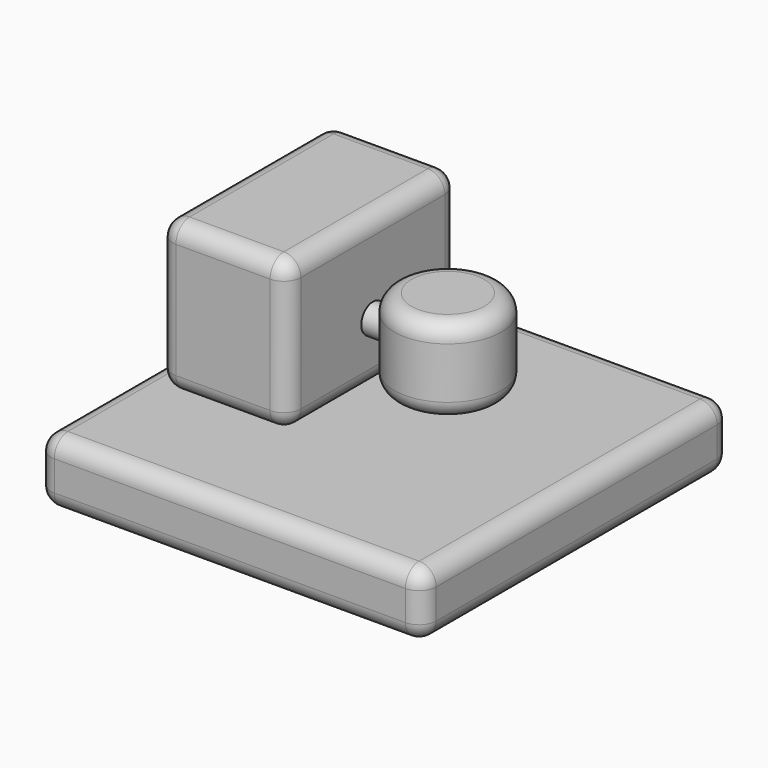
from build123d import *

# Parameters (mm, degrees)
F1_DEPTH      = 57.15
F2_DEPTH      = 57.15
F3_DEPTH      = 31.75
F4_DEPTH      = 31.75
F0_W          = 15.875
F0_H          = 25.4
F6_DEPTH      = 12.7
F7_DEPTH      = 12.7
F0_W_2        = 6.35
F0_H_2        = 4.318
F9_R          = 5.08
F10_R         = 5.08
F11_R         = 5.08
F12_R         = 5.08
F13_R         = 5.08
F13_2_R       = 5.08
F14_R         = 5.08
F15_R         = 5.08
F15_2_R       = 5.08
F16_R         = 5.08
F17_R         = 5.08
F18_R         = 5.08
F19_R         = 5.08
F20_T1_DEPTH  = 53.34
F20_S5_W      = 5.08
F20_S5_H      = 5.08
F20_T6_DEPTH  = 5.08
F20_S11_W     = 5.08
F20_S11_H     = 5.08
F20_T12_DEPTH = 5.08
F20_S17_W     = 5.08
F20_S17_H     = 5.08
F20_T18_DEPTH = 5.08
F20_S23_W     = 5.08
F20_S23_H     = 5.08
F20_T24_DEPTH = 5.08
F21_T1_DEPTH  = 53.34
F21_S5_W      = 5.08
F21_S5_H      = 5.08
F21_T6_DEPTH  = 5.08
F21_S11_W     = 5.08
F21_S11_H     = 5.08
F21_T12_DEPTH = 5.08
F21_S17_W     = 5.08
F21_S17_H     = 5.08
F21_T18_DEPTH = 5.08
F21_S23_W     = 5.08
F21_S23_H     = 5.08
F21_T24_DEPTH = 5.08


# Not quite as in the source:
# - a fillet or chamfer that OpenCascade refuses, or shapes differently, is made with other operations: its cross-section is extruded or revolved along the edge and cut away or added


with BuildPart() as f1:
    # F0 (on Front) → F1 (new body)
    with BuildSketch(Plane.XZ):
        Polygon((57.15, -57.15), (57.15, -38.1), (-22.337236915, -38.1), (-57.15, -38.1), (-57.15, -57.15), align=None)
    extrude(amount=F1_DEPTH)

    # F2 (add): a face of the model
    f2_faces = [f1.faces().sort_by_distance(p)[0] for p in [
        (0, 0, -47.625),
    ]]
    extrude(f2_faces, amount=F2_DEPTH)

    # F9
    f9_edges = [f1.edges().sort_by_distance(p)[0] for p in [
        (0, -57.15, -38.1),
    ]]
    fillet(f9_edges, radius=F9_R)

    # F10
    f10_edges = [f1.edges().sort_by_distance(p)[0] for p in [
        (-57.15, -57.15, -50.165),
    ]]
    fillet(f10_edges, radius=F10_R)

    # F11
    f11_edges = [f1.edges().sort_by_distance(p)[0] for p in [
        (2.54, -57.15, -57.15),
    ]]
    fillet(f11_edges, radius=F11_R)

    # F12
    f12_edges = [f1.edges().sort_by_distance(p)[0] for p in [
        (57.15, -57.15, -47.625),
    ]]
    fillet(f12_edges, radius=F12_R)

    # F14
    f14_edges = [f1.edges().sort_by_distance(p)[0] for p in [
        (0, 57.15, -38.1),
    ]]
    fillet(f14_edges, radius=F14_R)


with BuildPart() as f3:
    # F0 (on Front) → F3 (new body)
    with BuildSketch(Plane.XZ):
        Polygon((-41.387236915, -31.75), (-22.337236915, -31.75), (-3.287236915, -31.75), (-3.287236915, -18.161), (-3.287236915, -13.843), (-3.287236915, -9.525), (-3.287236915, 12.7), (-41.387236915, 12.7), (-41.387236915, -9.525), align=None)
    extrude(amount=F3_DEPTH)

    # F0 (on Front) → F4 (join)
    with BuildSketch(Plane.XZ):
        Polygon((-41.387236915, -31.75), (-22.337236915, -31.75), (-3.287236915, -31.75), (-3.287236915, -18.161), (-3.287236915, -13.843), (-3.287236915, -9.525), (-3.287236915, 12.7), (-41.387236915, 12.7), (-41.387236915, -9.525), align=None)
    extrude(amount=-F4_DEPTH)

    # F16
    f16_edges = [f3.edges().sort_by_distance(p)[0] for p in [
        (-41.387237, -31.75, -9.525),
        (-22.337237, -31.75, 12.7),
        (-3.287237, -31.75, -9.525),
        (-22.337237, -31.75, -31.75),
    ]]
    fillet(f16_edges, radius=F16_R)

    # F19
    f19_edges = [f3.edges().sort_by_distance(p)[0] for p in [
        (-22.337237, 31.75, 12.7),
        (-41.387237, 31.75, -9.525),
        (-22.337237, 31.75, -31.75),
        (-3.287237, 31.75, -9.525),
    ]]
    fillet(f19_edges, radius=F19_R)

    # F20: fillet of radius 5.08 on 2 edges, made by hand

    # F20_s2 → F20_t1 (cut)
    with BuildSketch(Plane.XZ.offset(-26.67)):
        with BuildLine():
            ThreePointArc((-3.287236915, 7.62), (-4.7751344666, 11.2121024484), (-8.367236915, 12.7))
            Line((-8.367236915, 12.7), (-3.287236915, 12.7))
            Line((-3.287236915, 12.7), (-3.287236915, 7.62))
        make_face()
        with BuildLine():
            ThreePointArc((-41.387236915, 7.62), (-39.8993393635, 11.2121024484), (-36.307236915, 12.7))
            Line((-36.307236915, 12.7), (-41.387236915, 12.7))
            Line((-41.387236915, 12.7), (-41.387236915, 7.62))
        make_face()
    extrude(amount=F20_T1_DEPTH, mode=Mode.SUBTRACT)


with BuildPart() as f5:
    # F0 (on Front) → F5 (revolve)
    with BuildSketch(Plane.XZ):
        with Locations((26.875263085, -12.7)):
            Rectangle(F0_W, F0_H)
    revolve(axis=Axis((18.937763085, 0, -12.7), (0, 0, -1)))

    # F17
    f17_edges = [f5.edges().sort_by_distance(p)[0] for p in [
        (3.062763, 0, 0),
    ]]
    fillet(f17_edges, radius=F17_R)

    # F18
    f18_edges = [f5.edges().sort_by_distance(p)[0] for p in [
        (3.062763, 0, -25.4),
    ]]
    fillet(f18_edges, radius=F18_R)


with BuildPart() as f6:
    # F0 (on Front) → F6 (new body)
    with BuildSketch(Plane.XZ):
        with BuildLine():
            Line((-57.15, -38.1), (-22.337236915, -38.1))
            Line((-22.337236915, -38.1), (-22.337236915, -31.75))
            Line((-22.337236915, -31.75), (-41.387236915, -31.75))
            Line((-41.387236915, -31.75), (-41.387236915, -9.525))
            ThreePointArc((-41.387236915, -9.525), (-52.9479711415, -21.7828669409), (-57.15, -38.1))
        make_face()
    extrude(amount=F6_DEPTH)

    # F13
    f13_edges = [f6.edges().sort_by_distance(p)[0] for p in [
        (-57.15, -6.35, -38.1),
    ]]
    fillet(f13_edges, radius=F13_R)

    # F15
    f15_edges = [f6.edges().sort_by_distance(p)[0] for p in [
        (-51.381264, -12.7, -19.219307),
    ]]
    fillet(f15_edges, radius=F15_R)


with BuildPart() as f7:
    # F0 (on Front) → F7 (new body)
    with BuildSketch(Plane.XZ):
        with BuildLine():
            Line((-57.15, -38.1), (-22.337236915, -38.1))
            Line((-22.337236915, -38.1), (-22.337236915, -31.75))
            Line((-22.337236915, -31.75), (-41.387236915, -31.75))
            Line((-41.387236915, -31.75), (-41.387236915, -9.525))
            ThreePointArc((-41.387236915, -9.525), (-52.9479711415, -21.7828669409), (-57.15, -38.1))
        make_face()
    extrude(amount=-F7_DEPTH)

    # F13#2
    f13_2_edges = [f7.edges().sort_by_distance(p)[0] for p in [
        (-57.15, 6.35, -38.1),
    ]]
    fillet(f13_2_edges, radius=F13_2_R)

    # F15#2
    f15_2_edges = [f7.edges().sort_by_distance(p)[0] for p in [
        (-51.381264, 12.7, -19.219307),
    ]]
    fillet(f15_2_edges, radius=F15_2_R)


with BuildPart() as f8:
    # F0 (on Front) → F8 (revolve)
    with BuildSketch(Plane.XZ):
        with Locations((-0.112236915, -16.002)):
            Rectangle(F0_W_2, F0_H_2)
    revolve(axis=Axis((-0.112236915, 0, -13.843), (1, 0, 0)))


with BuildPart() as f20_tool4:
    # F20_s5 → F20_t6 (new body)
    with BuildSketch(Plane.YZ.offset(-36.307236915)):
        with Locations((-29.21, 10.16)):
            Rectangle(F20_S5_W, F20_S5_H)
    extrude(amount=-F20_T6_DEPTH)

    # F20_s7 → F20_t8 (revolve, cut)
    with BuildSketch(Plane(origin=(-36.307236915, -26.67, 7.62), x_dir=(0, 0.7071067812, -0.7071067812), z_dir=(0, 0.7071067812, 0.7071067812))):
        with BuildLine():
            ThreePointArc((0, -5.08), (5.08, 0), (0, 5.08))
            Line((0, 5.08), (0, -5.08))
        make_face()
    revolve(axis=Axis((-36.307236915, -26.67, 7.62), (-1, 0, 0)), mode=Mode.SUBTRACT)


with BuildPart() as f3_1:
    add(f3.part)

    # F20_t3: cut F20_tool4
    add(f20_tool4.part, mode=Mode.SUBTRACT)


with BuildPart() as f20_tool10:
    # F20_s11 → F20_t12 (new body)
    with BuildSketch(Plane.YZ.offset(-36.307236915)):
        with Locations((29.21, 10.16)):
            Rectangle(F20_S11_W, F20_S11_H)
    extrude(amount=-F20_T12_DEPTH)

    # F20_s13 → F20_t14 (revolve, cut)
    with BuildSketch(Plane(origin=(-36.307236915, 26.67, 7.62), x_dir=(0, -0.7071067812, -0.7071067812), z_dir=(0, 0.7071067812, -0.7071067812))):
        with BuildLine():
            ThreePointArc((0, -5.08), (5.08, 0), (0, 5.08))
            Line((0, 5.08), (0, -5.08))
        make_face()
    revolve(axis=Axis((-36.307236915, 26.67, 7.62), (-1, 0, 0)), mode=Mode.SUBTRACT)


with BuildPart() as f3_2:
    add(f3_1.part)

    # F20_t9: cut F20_tool10
    add(f20_tool10.part, mode=Mode.SUBTRACT)


with BuildPart() as f20_tool16:
    # F20_s17 → F20_t18 (new body)
    with BuildSketch(Plane.YZ.offset(-8.367236915)):
        with Locations((29.21, 10.16)):
            Rectangle(F20_S17_W, F20_S17_H)
    extrude(amount=F20_T18_DEPTH)

    # F20_s19 → F20_t20 (revolve, cut)
    with BuildSketch(Plane(origin=(-8.367236915, 26.67, 7.62), x_dir=(0, -0.7071067812, -0.7071067812), z_dir=(0, -0.7071067812, 0.7071067812))):
        with BuildLine():
            ThreePointArc((0, -5.08), (5.08, 0), (0, 5.08))
            Line((0, 5.08), (0, -5.08))
        make_face()
    revolve(axis=Axis((-8.367236915, 26.67, 7.62), (1, 0, 0)), mode=Mode.SUBTRACT)


with BuildPart() as f3_3:
    add(f3_2.part)

    # F20_t15: cut F20_tool16
    add(f20_tool16.part, mode=Mode.SUBTRACT)


with BuildPart() as f20_tool22:
    # F20_s23 → F20_t24 (new body)
    with BuildSketch(Plane.YZ.offset(-8.367236915)):
        with Locations((-29.21, 10.16)):
            Rectangle(F20_S23_W, F20_S23_H)
    extrude(amount=F20_T24_DEPTH)

    # F20_s25 → F20_t26 (revolve, cut)
    with BuildSketch(Plane(origin=(-8.367236915, -26.67, 7.62), x_dir=(0, 0.7071067812, -0.7071067812), z_dir=(0, -0.7071067812, -0.7071067812))):
        with BuildLine():
            ThreePointArc((0, -5.08), (5.08, 0), (0, 5.08))
            Line((0, 5.08), (0, -5.08))
        make_face()
    revolve(axis=Axis((-8.367236915, -26.67, 7.62), (1, 0, 0)), mode=Mode.SUBTRACT)


with BuildPart() as f3_4:
    add(f3_3.part)

    # F20_t21: cut F20_tool22
    add(f20_tool22.part, mode=Mode.SUBTRACT)

    # F21: fillet of radius 5.08 on 2 edges, made by hand

    # F21_s2 → F21_t1 (cut)
    with BuildSketch(Plane.XZ.offset(-26.67)):
        with BuildLine():
            ThreePointArc((-8.367236915, -31.75), (-4.7751344666, -30.2621024484), (-3.287236915, -26.67))
            Line((-3.287236915, -26.67), (-3.287236915, -31.75))
            Line((-3.287236915, -31.75), (-8.367236915, -31.75))
        make_face()
        with BuildLine():
            ThreePointArc((-36.307236915, -31.75), (-39.8993393635, -30.2621024484), (-41.387236915, -26.67))
            Line((-41.387236915, -26.67), (-41.387236915, -31.75))
            Line((-41.387236915, -31.75), (-36.307236915, -31.75))
        make_face()
    extrude(amount=F21_T1_DEPTH, mode=Mode.SUBTRACT)


with BuildPart() as f21_tool4:
    # F21_s5 → F21_t6 (new body)
    with BuildSketch(Plane.XY.offset(-26.67)):
        with Locations((-38.847236915, -29.21)):
            Rectangle(F21_S5_W, F21_S5_H)
    extrude(amount=-F21_T6_DEPTH)

    # F21_s7 → F21_t8 (revolve, cut)
    with BuildSketch(Plane(origin=(-36.307236915, -26.67, -26.67), x_dir=(0.7071067812, 0.7071067812, 0), z_dir=(-0.7071067812, 0.7071067812, 0))):
        with BuildLine():
            ThreePointArc((0, -5.08), (5.08, 0), (0, 5.08))
            Line((0, 5.08), (0, -5.08))
        make_face()
    revolve(axis=Axis((-36.307236915, -26.67, -26.67), (0, 0, -1)), mode=Mode.SUBTRACT)


with BuildPart() as f3_5:
    add(f3_4.part)

    # F21_t3: cut F21_tool4
    add(f21_tool4.part, mode=Mode.SUBTRACT)


with BuildPart() as f21_tool10:
    # F21_s11 → F21_t12 (new body)
    with BuildSketch(Plane.XY.offset(-26.67)):
        with Locations((-38.847236915, 29.21)):
            Rectangle(F21_S11_W, F21_S11_H)
    extrude(amount=-F21_T12_DEPTH)

    # F21_s13 → F21_t14 (revolve, cut)
    with BuildSketch(Plane(origin=(-36.307236915, 26.67, -26.67), x_dir=(0.7071067812, -0.7071067812, 0), z_dir=(0.7071067812, 0.7071067812, 0))):
        with BuildLine():
            ThreePointArc((0, -5.08), (5.08, 0), (0, 5.08))
            Line((0, 5.08), (0, -5.08))
        make_face()
    revolve(axis=Axis((-36.307236915, 26.67, -26.67), (0, 0, -1)), mode=Mode.SUBTRACT)


with BuildPart() as f3_6:
    add(f3_5.part)

    # F21_t9: cut F21_tool10
    add(f21_tool10.part, mode=Mode.SUBTRACT)


with BuildPart() as f21_tool16:
    # F21_s17 → F21_t18 (new body)
    with BuildSketch(Plane.XY.offset(-26.67)):
        with Locations((-5.827236915, 29.21)):
            Rectangle(F21_S17_W, F21_S17_H)
    extrude(amount=-F21_T18_DEPTH)

    # F21_s19 → F21_t20 (revolve, cut)
    with BuildSketch(Plane(origin=(-8.367236915, 26.67, -26.67), x_dir=(-0.7071067812, -0.7071067812, 0), z_dir=(0.7071067812, -0.7071067812, 0))):
        with BuildLine():
            ThreePointArc((0, -5.08), (5.08, 0), (0, 5.08))
            Line((0, 5.08), (0, -5.08))
        make_face()
    revolve(axis=Axis((-8.367236915, 26.67, -26.67), (0, 0, -1)), mode=Mode.SUBTRACT)


with BuildPart() as f3_7:
    add(f3_6.part)

    # F21_t15: cut F21_tool16
    add(f21_tool16.part, mode=Mode.SUBTRACT)


with BuildPart() as f21_tool22:
    # F21_s23 → F21_t24 (new body)
    with BuildSketch(Plane.XY.offset(-26.67)):
        with Locations((-5.827236915, -29.21)):
            Rectangle(F21_S23_W, F21_S23_H)
    extrude(amount=-F21_T24_DEPTH)

    # F21_s25 → F21_t26 (revolve, cut)
    with BuildSketch(Plane(origin=(-8.367236915, -26.67, -26.67), x_dir=(-0.7071067812, 0.7071067812, 0), z_dir=(-0.7071067812, -0.7071067812, 0))):
        with BuildLine():
            ThreePointArc((0, -5.08), (5.08, 0), (0, 5.08))
            Line((0, 5.08), (0, -5.08))
        make_face()
    revolve(axis=Axis((-8.367236915, -26.67, -26.67), (0, 0, -1)), mode=Mode.SUBTRACT)


with BuildPart() as f3_8:
    add(f3_7.part)

    # F21_t21: cut F21_tool22
    add(f21_tool22.part, mode=Mode.SUBTRACT)


solid = Compound([f1.part, f5.part, f6.part, f7.part, f8.part, f3_8.part])
